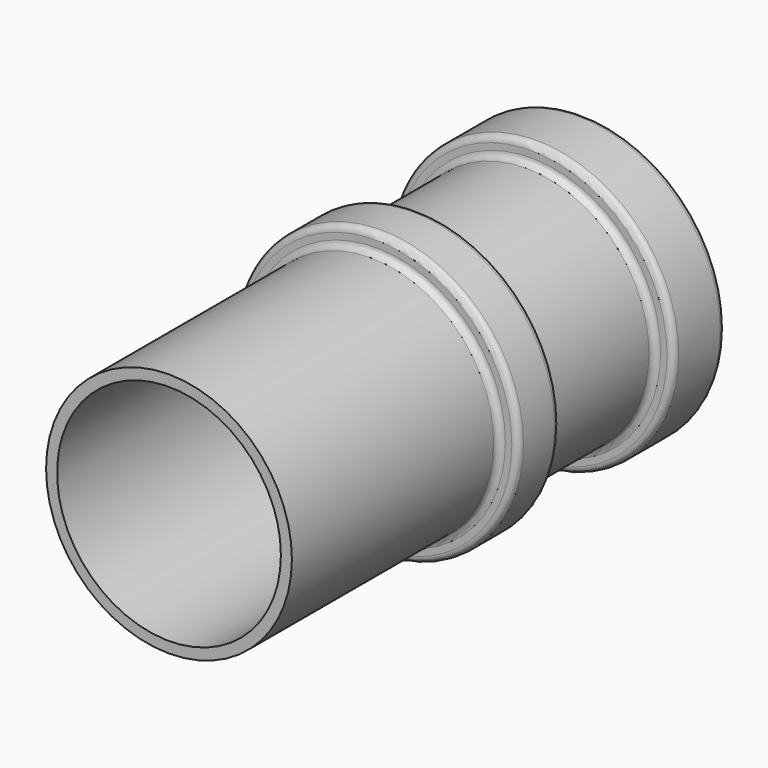
from build123d import *

# Parameters (mm, degrees)
F0_R     = 9.5
F0_R_2   = 8.65
F1_DEPTH = 40
F0_R_3   = 11
F2_DEPTH = 20
F3_DEPTH = 16
F4_R     = 11
F4_R_2   = 9.5
F5_DEPTH = 5
F6_R     = 0.5
F4_R_3   = 8.65
F4_R_4   = 8.2
F7_DEPTH = 1.5
F8_DEPTH = 1


# Not quite as in the source:
# - a fillet or chamfer that OpenCascade refuses, or shapes differently, is made with other operations: its cross-section is extruded or revolved along the edge and cut away or added


with BuildPart() as f1:
    # F0 (on Front) → F1 (new body)
    with BuildSketch(Plane.XZ):
        Circle(F0_R)
        Circle(F0_R_2, mode=Mode.SUBTRACT)
    extrude(amount=F1_DEPTH)

    # F0 (on Front) → F2 (join)
    with BuildSketch(Plane.XZ):
        Circle(F0_R_3)
        Circle(F0_R, mode=Mode.SUBTRACT)
    extrude(amount=F2_DEPTH)

    # F0 (on Front) → F3 (cut)
    with BuildSketch(Plane.XZ):
        Circle(F0_R_3)
        Circle(F0_R, mode=Mode.SUBTRACT)
    extrude(amount=F3_DEPTH, mode=Mode.SUBTRACT)

    # F4 (on face) → F5 (join)
    with BuildSketch(Plane.XZ):
        Circle(F4_R)
        Circle(F4_R_2, mode=Mode.SUBTRACT)
    extrude(amount=F5_DEPTH)

    # F6
    f6_edges = [f1.edges().sort_by_distance(p)[0] for p in [
        (-11, 0, 0),
        (-11, -5, 0),
        (-11, -16, 0),
        (-11, -20, 0),
        (-9.5, -5, 0),
        (-9.5, -16, 0),
        (-9.5, -20, 0),
    ]]
    fillet(f6_edges, radius=F6_R)

    # F4 (on face) → F7 (join)
    with BuildSketch(Plane.XZ):
        Circle(F4_R_3)
        Circle(F4_R_4, mode=Mode.SUBTRACT)
        Circle(F4_R_4)
    extrude(amount=F7_DEPTH)

    # F4 (on face) → F8 (join)
    with BuildSketch(Plane.XZ):
        Circle(F4_R_3)
        Circle(F4_R_4, mode=Mode.SUBTRACT)
        Circle(F4_R_4)
    extrude(amount=-F8_DEPTH)

    # F9: fillet of radius 1.5 on 1 edges, made by hand

    # F9_s1 → F9_t2 (revolve, cut)
    with BuildSketch(Plane.XY):
        with BuildLine():
            ThreePointArc((8.65, 0), (8.1018118414, 0.7247448714), (7.2357864376, 1))
            Line((7.2357864376, 1), (8.65, 1))
            Line((8.65, 1), (8.65, 0))
        make_face()
    revolve(axis=Axis((0, 1, 0), (0, -1, 0)), mode=Mode.SUBTRACT)


solid = f1.part
